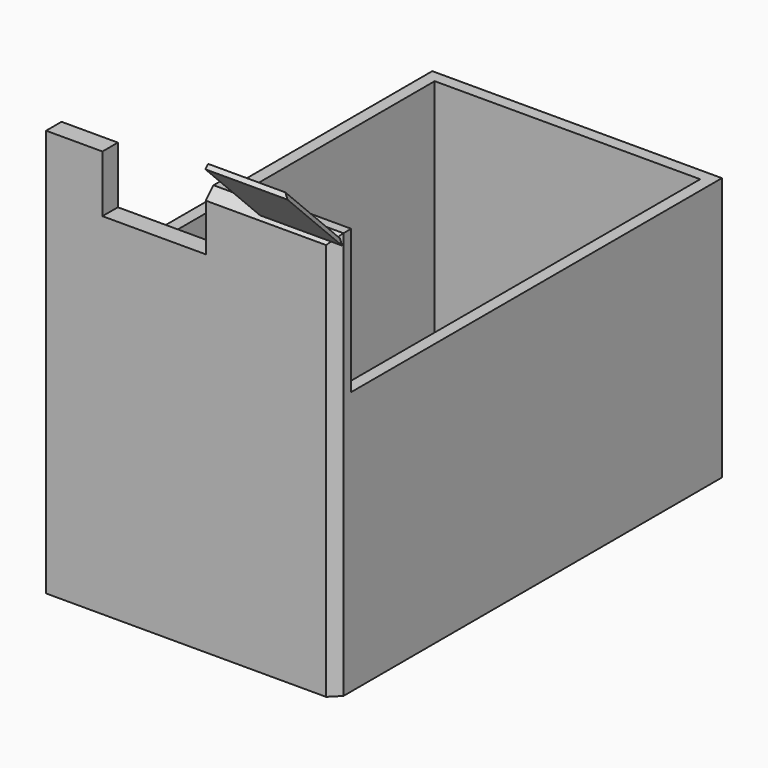
from build123d import *

# Parameters (mm, degrees)
F0_W         = 76.2
F0_H         = 127
F1_DEPTH     = 69.342
F3_DEPTH     = 5.08
F4_T         = -3.175
F7_SIZE      = 2.54
F8_W         = 25.4
F8_H         = 1.27
F9_DEPTH     = 25.4
F10_T1_DEPTH = 38.4641495789


# Not quite as in the source:
# - a fillet or chamfer that OpenCascade refuses, or shapes differently, is made with other operations: its cross-section is extruded or revolved along the edge and cut away or added
# - a feature of the source that left no trace in its solid (it failed there, or was rolled back) is left out


with BuildPart() as f1:
    # F0 (on Top) → F1 (new body)
    with BuildSketch(Plane.XY):
        with Locations((38.1, 63.5)):
            Rectangle(F0_W, F0_H)
    extrude(amount=F1_DEPTH)

    # F2 (on face) → F3 (join)
    with BuildSketch(Plane.XZ):
        Polygon((0, 107.1759281516), (0, 69.342), (76.2, 69.342), (76.2, 107.1759281516), (42.011950165, 107.1759281516), (42.011950165, 92.1983985066), (14.8228770122, 92.1983985066), (14.8228770122, 107.1759281516), align=None)
    extrude(amount=-F3_DEPTH)

    # F4: a shell. OpenCascade refuses it in one call, so the cavity is built on its own and cut out:
    # the body offset inwards by the wall thickness, plus a prism from it out through each open face.
    f4_core = offset(f1.part, amount=F4_T, kind=Kind.INTERSECTION, mode=Mode.PRIVATE)
    f4_exits = [f4_core.faces().sort_by_distance(p)[0] for p in [
        (38.1, 63.5, 66.167),
    ]]
    add(f4_core, mode=Mode.SUBTRACT)
    extrude(f4_exits, amount=-F4_T, mode=Mode.SUBTRACT)

    # F7
    f7_edges = [f1.edges().sort_by_distance(p)[0] for p in [
        (59.105975, 0, 107.175928),
        (76.2, 0, 53.587964),
    ]]
    chamfer(f7_edges, length=F7_SIZE)

    # F8 (on face) → F9 (join)
    with BuildSketch(Plane(origin=(0, -52.3179640758, 52.3179640758), x_dir=(1, 0, 0), z_dir=(0, -0.7071067812, 0.7071067812))):
        with Locations((68.3882001948, 75.6758768002)):
            Rectangle(F8_W, F8_H)
    extrude(amount=F9_DEPTH)

    # F10: chamfer of 5.08 on 1 edges, made by hand

    # F10_s2 → F10_t1 (cut)
    with BuildSketch(Plane(origin=(0, -52.3179640758, 52.3179640758), x_dir=(1, 0, 0), z_dir=(0, -0.7071067812, 0.7071067812))):
        Polygon((76.0082001948, 76.3108768002), (81.0882001948, 71.2308768002), (81.0882001948, 76.3108768002), align=None)
    extrude(amount=F10_T1_DEPTH, mode=Mode.SUBTRACT)


solid = f1.part
